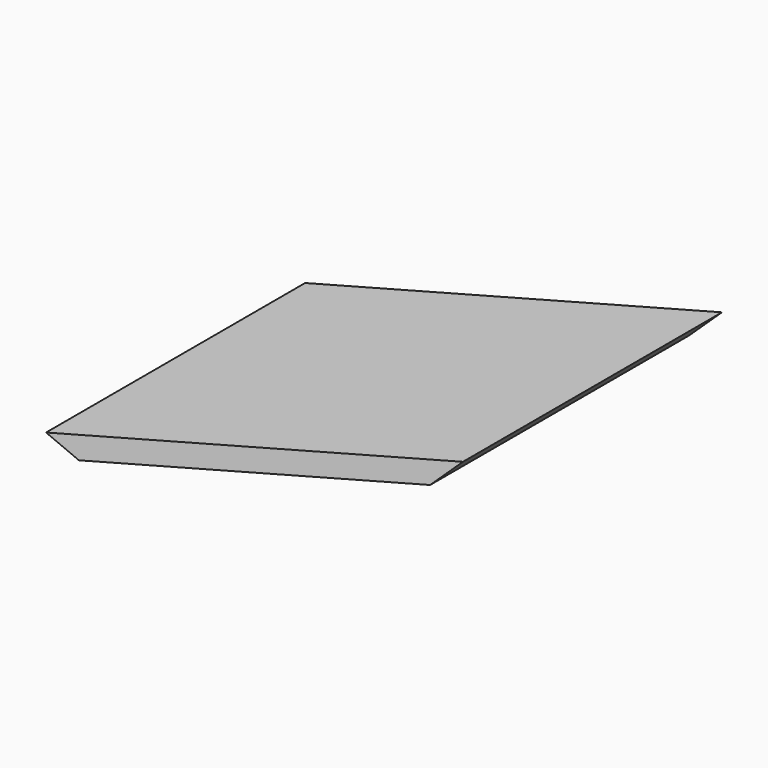
from build123d import *

# Parameters (mm, degrees)
F1_DEPTH = 19.05
F2_SIZE  = 19.04999


# Not quite as in the source:
# - a fillet or chamfer is up to 0.001 mm smaller than in the source, because OpenCascade refuses the exact size


with BuildPart() as f1:
    # F0 (on Top) → F1 (new body)
    with BuildSketch(Plane.XY):
        Polygon((-120.9837489087, -207.2259), (120.9837489087, -67.5259), (120.9837489087, 207.2259), (-120.9837489087, 67.5259), align=None)
    extrude(amount=F1_DEPTH)

    # F2 (size 19.05 in the source; OpenCascade refuses exactly that, so slightly less here)
    f2_edges = [f1.edges().sort_by_distance(p)[0] for p in [
        (-120.983749, -69.85, 0),
        (120.983749, 69.85, 0),
    ]]
    chamfer(f2_edges, length=F2_SIZE)


solid = f1.part
